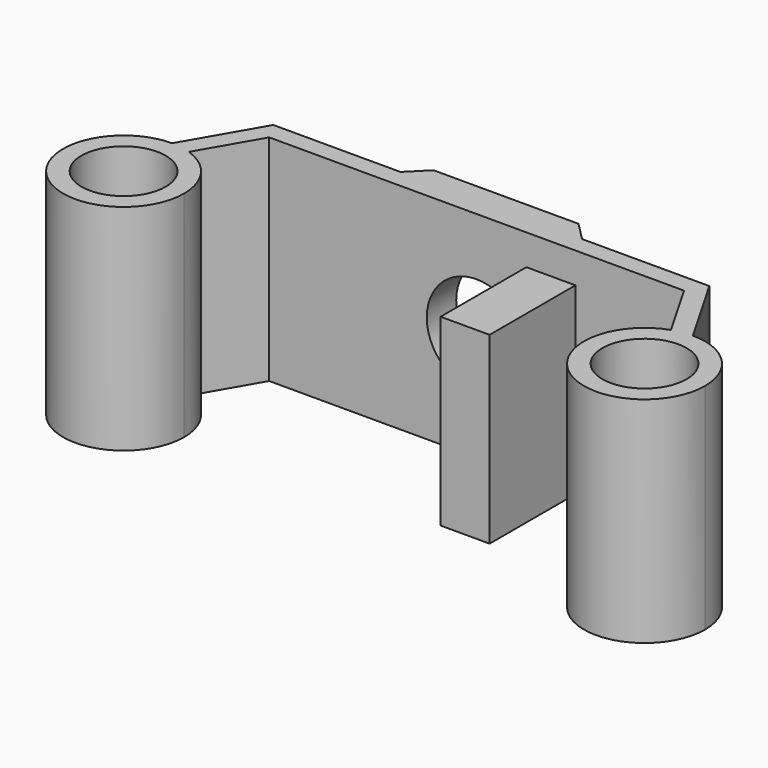
from build123d import *

# Parameters (mm, degrees)
F0_R     = 2.75
F0_W     = 9.4574374158
F0_H     = 1.2
F1_DEPTH = 14
F2_R     = 3.25
F3_DEPTH = 54
F4_DEPTH = 25
F5_SIZE  = 1.19999
F7_DEPTH = 7


# Not quite as in the source:
# - a fillet or chamfer is up to 0.001 mm smaller than in the source, because OpenCascade refuses the exact size


with BuildPart() as f1:
    # F0 (on Top) → F1 (new body)
    with BuildSketch(Plane.XY):
        with BuildLine():
            ThreePointArc((0, 3.95), (-2.7930717857, -2.7930717857), (3.95, 0))
            ThreePointArc((3.95, 0), (3.2094391954, 2.302607229), (1.2654430121, 3.7418115911))
            ThreePointArc((1.2654430121, 3.7418115911), (0.6412270328, 3.8976054049), (0, 3.95))
        make_face()
        Circle(F0_R, mode=Mode.SUBTRACT)
        with BuildLine():
            ThreePointArc((0, 3.95), (0.6412270328, 3.8976054049), (1.2654430121, 3.7418115911))
            Line((1.2654430121, 3.7418115911), (3.4641016151, 7.55))
            Line((3.4641016151, 7.55), (30.5358983849, 7.55))
            Line((30.5358983849, 7.55), (32.7345569879, 3.7418115911))
            ThreePointArc((32.7345569879, 3.7418115911), (33.3587729672, 3.8976054049), (34, 3.95))
            Line((34, 3.95), (31.2287187079, 8.75))
            Line((31.2287187079, 8.75), (21.7287187079, 8.75))
            Line((21.7287187079, 8.75), (12.2712812921, 8.75))
            Line((12.2712812921, 8.75), (2.7712812921, 8.75))
            Line((2.7712812921, 8.75), (0, 3.95))
        make_face()
        with Locations((17, 9.35)):
            Rectangle(F0_W, F0_H)
        with BuildLine():
            ThreePointArc((34, 3.95), (33.3587729672, 3.8976054049), (32.7345569879, 3.7418115911))
            ThreePointArc((32.7345569879, 3.7418115911), (31.697392771, -3.2094391954), (37.95, 0))
            ThreePointArc((37.95, 0), (36.7930717857, 2.7930717857), (34, 3.95))
        make_face()
        with Locations((34, 0)):
            Circle(F0_R, mode=Mode.SUBTRACT)
    extrude(amount=F1_DEPTH)

    # F2 (on face) → F3 (cut)
    with BuildSketch(Plane(origin=(0, 8.75, 0), x_dir=(-1, 0, 0), z_dir=(0, 1, 0))):
        with Locations((-17, 7)):
            Circle(F2_R)
    extrude(amount=-F3_DEPTH, mode=Mode.SUBTRACT)

    # F4 (cut): a face of the model
    f4_faces = [f1.faces().sort_by_distance(p)[0] for p in [
        (17, 8.75, 7),
    ]]
    extrude(f4_faces, amount=-F4_DEPTH, mode=Mode.SUBTRACT)

    # F5 (size 1.2 in the source; OpenCascade refuses exactly that, so slightly less here)
    f5_edges = [f1.edges().sort_by_distance(p)[0] for p in [
        (21.728719, 8.75, 7),
        (12.271281, 8.75, 7),
    ]]
    chamfer(f5_edges, length=F5_SIZE)

    # F6 (on face) → F7 (join)
    with BuildSketch(Plane.XZ.offset(-7.55)):
        Polygon((20.25, 0), (23.45, 0), (23.45, 12), (20.25, 12), (20.25, 7), align=None)
    extrude(amount=F7_DEPTH)


solid = f1.part
